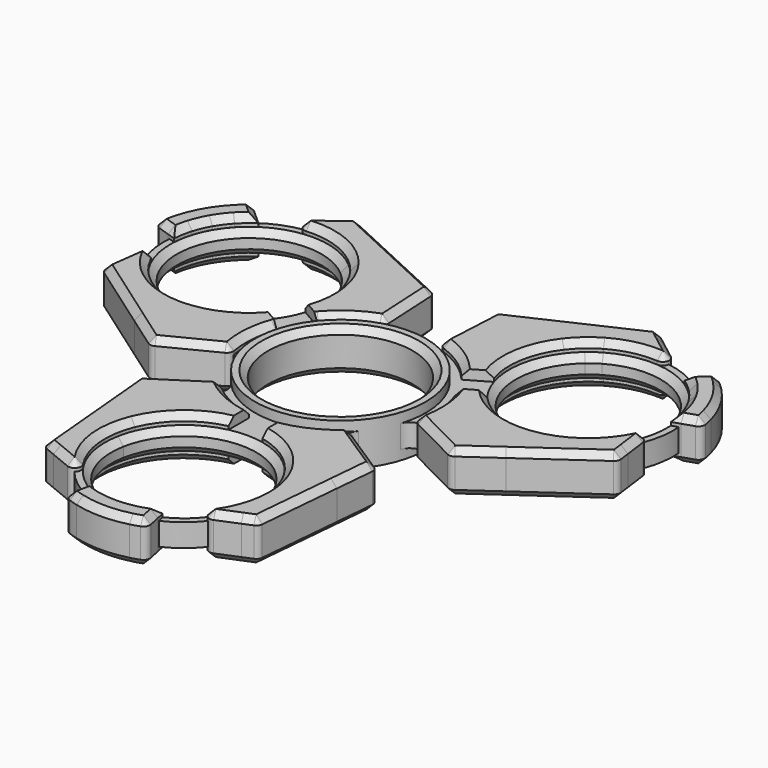
from build123d import *

# Parameters (mm, degrees)
F0_R         = 13.1
F0_R_2       = 11.1
F1_DEPTH     = 6.5
F3_DEPTH     = 6.5
F4_R         = 1
F4_2_R       = 1
F4_3_R       = 1
F6_SIZE      = 1
F6_2_SIZE    = 1
F6_3_SIZE    = 1
F6_4_SIZE    = 1
F7_COUNT     = 3
F10_DEPTH    = 3.5
F11_SIZE     = 1
F12_COUNT    = 3
F14_T1_DEPTH = 3.5


# Not quite as in the source:
# - a fillet or chamfer that OpenCascade refuses, or shapes differently, is made with other operations: its cross-section is extruded or revolved along the edge and cut away or added
# - two fillets or chamfers of one size are made in one step


with BuildPart() as f1:
    # F0 (on Top) → F1 (new body)
    with BuildSketch(Plane.XY):
        Circle(F0_R)
        Circle(F0_R_2, mode=Mode.SUBTRACT)
    extrude(amount=F1_DEPTH)

    # F6
    f6_edges = [f1.edges().sort_by_distance(p)[0] for p in [
        (-11.1, 0, 6.5),
        (-11.1, 0, 0),
    ]]
    chamfer(f6_edges, length=F6_SIZE)


with BuildPart() as f3:
    # F2 (on Top) → F3 (new body)
    with BuildSketch(Plane.XY):
        with BuildLine():
            Line((-14.7820725202, -23.8770650822), (-11.1789423434, -25.3695304684))
            ThreePointArc((-11.1789423434, -25.3695304684), (-7.7703064339, -20.7246381244), (-2.6, -18.1826398887))
            Line((-2.6, -18.1826398887), (-2.6, -14.2649921136))
            ThreePointArc((-2.6, -14.2649921136), (-2.6733155154, -14.2514344596), (-2.7465603489, -14.2375))
            ThreePointArc((-2.7465603489, -14.2375), (-10.0021770784, -17.5117473723), (-14.7820725202, -23.8770650822))
        make_face()
        with BuildLine():
            ThreePointArc((-6.2404261974, -40.3666330539), (-11.4929052715, -33.7845909184), (-11.1789423434, -25.3695304684))
            Line((-11.1789423434, -25.3695304684), (-14.7820725202, -23.8770650822))
            ThreePointArc((-14.7820725202, -23.8770650822), (-15.9929194856, -30.4759478198), (-14.3917986532, -36.9911466532))
            Line((-14.3917986532, -36.9911466532), (-6.2404261974, -40.3666330539))
        make_face()
        with BuildLine():
            Line((-17.6223396977, -22.7005878965), (-14.7820725202, -23.8770650822))
            ThreePointArc((-14.7820725202, -23.8770650822), (-10.0021770784, -17.5117473723), (-2.7465603489, -14.2375))
            ThreePointArc((-2.7465603489, -14.2375), (-6.5777497188, -12.9221982896), (-9.8956077284, -10.5984408139))
            Line((-9.8956077284, -10.5984408139), (-18.2283200336, -16.0097674569))
            Line((-18.2283200336, -16.0097674569), (-17.6223396977, -22.7005878965))
        make_face()
        with BuildLine():
            ThreePointArc((-14.3917986532, -36.9911466532), (-15.9929194856, -30.4759478198), (-14.7820725202, -23.8770650822))
            Line((-14.7820725202, -23.8770650822), (-17.6223396977, -22.7005878965))
            Line((-17.6223396977, -22.7005878965), (-16.4035077071, -36.1580971771))
            Line((-16.4035077071, -36.1580971771), (-14.3917986532, -36.9911466532))
        make_face()
    extrude(amount=F3_DEPTH)

    # F4#2
    f4_2_edges = [f3.edges().sort_by_distance(p)[0] for p in [
        (-6.240426, -40.366633, 3.25),
        (-9.895608, -10.598441, 3.25),
        (-18.22832, -16.009767, 3.25),
        (-16.403508, -36.158097, 3.25),
    ]]
    fillet(f4_2_edges, radius=F4_2_R)

    # F6#2
    f6_2_edges = [f3.edges().sort_by_distance(p)[0] for p in [
        (-11.248136, -25.540243, 6.5),
        (-11.248136, -25.540243, 0),
    ]]
    chamfer(f6_2_edges, length=F6_2_SIZE)


with BuildPart() as f3b:
    # F2 (on Top) → F3, piece 2 (new body)
    with BuildSketch(Plane.XY):
        with BuildLine():
            Line((14.7820725202, -23.8770650822), (11.1789423434, -25.3695304684))
            ThreePointArc((11.1789423434, -25.3695304684), (11.8675018929, -27.6394071036), (12.1, -30))
            ThreePointArc((12.1, -30), (10.5337352584, -35.9540256554), (6.2404261974, -40.3666330539))
            Line((6.2404261974, -40.3666330539), (14.3917986532, -36.9911466532))
            ThreePointArc((14.3917986532, -36.9911466532), (15.5927672087, -33.5868664283), (16, -30))
            ThreePointArc((16, -30), (15.6925644865, -26.8785548477), (14.7820725202, -23.8770650822))
        make_face()
        with BuildLine():
            Line((17.6223396977, -22.7005878965), (14.7820725202, -23.8770650822))
            ThreePointArc((14.7820725202, -23.8770650822), (15.6925644865, -26.8785548477), (16, -30))
            ThreePointArc((16, -30), (15.5927672087, -33.5868664283), (14.3917986532, -36.9911466532))
            Line((14.3917986532, -36.9911466532), (16.4035077071, -36.1580971771))
            Line((16.4035077071, -36.1580971771), (17.6223396977, -22.7005878965))
        make_face()
        with BuildLine():
            ThreePointArc((2.7465603489, -14.2375), (10.0021770784, -17.5117473723), (14.7820725202, -23.8770650822))
            Line((14.7820725202, -23.8770650822), (17.6223396977, -22.7005878965))
            Line((17.6223396977, -22.7005878965), (18.2283200336, -16.0097674569))
            Line((18.2283200336, -16.0097674569), (9.8956077284, -10.5984408139))
            ThreePointArc((9.8956077284, -10.5984408139), (6.5777497188, -12.9221982896), (2.7465603489, -14.2375))
        make_face()
        with BuildLine():
            ThreePointArc((2.6, -18.1826398887), (7.7703064339, -20.7246381244), (11.1789423434, -25.3695304684))
            Line((11.1789423434, -25.3695304684), (14.7820725202, -23.8770650822))
            ThreePointArc((14.7820725202, -23.8770650822), (10.0021770784, -17.5117473723), (2.7465603489, -14.2375))
            ThreePointArc((2.7465603489, -14.2375), (2.6733155154, -14.2514344596), (2.6, -14.2649921136))
            Line((2.6, -14.2649921136), (2.6, -18.1826398887))
        make_face()
    extrude(amount=F3_DEPTH)

    # F4#3
    f4_3_edges = [f3b.edges().sort_by_distance(p)[0] for p in [
        (6.240426, -40.366633, 3.25),
        (16.403508, -36.158097, 3.25),
        (18.22832, -16.009767, 3.25),
        (9.895608, -10.598441, 3.25),
    ]]
    fillet(f4_3_edges, radius=F4_3_R)

    # F6#3
    f6_3_edges = [f3b.edges().sort_by_distance(p)[0] for p in [
        (11.248136, -25.540243, 6.5),
        (11.248136, -25.540243, 0),
    ]]
    chamfer(f6_3_edges, length=F6_3_SIZE)


with BuildPart() as f3c:
    # F2 (on Top) → F3, piece 3 (new body)
    with BuildSketch(Plane.XY):
        with BuildLine():
            Line((2.8440204456, -42.1), (0, -42.1))
            Line((0, -42.1), (-2.8440204456, -42.1))
            Line((-2.8440204456, -42.1), (-4.0641319608, -45.4752328385))
            ThreePointArc((-4.0641319608, -45.4752328385), (0, -46), (4.0641319608, -45.4752328385))
            Line((4.0641319608, -45.4752328385), (2.8440204456, -42.1))
        make_face()
        with BuildLine():
            Line((-2.8440204456, -42.1), (0, -42.1))
            ThreePointArc((0, -42.1), (-1.3744675345, -42.0216820369), (-2.7311424248, -41.7877419829))
            Line((-2.7311424248, -41.7877419829), (-2.8440204456, -42.1))
        make_face()
        with BuildLine():
            ThreePointArc((2.7311424248, -41.7877419829), (1.3744675345, -42.0216820369), (0, -42.1))
            Line((0, -42.1), (2.8440204456, -42.1))
            Line((2.8440204456, -42.1), (2.7311424248, -41.7877419829))
        make_face()
        with BuildLine():
            Line((-4.0641319608, -45.4752328385), (-2.8440204456, -42.1))
            Line((-2.8440204456, -42.1), (-5.6838904288, -42.1))
            Line((-5.6838904288, -42.1), (-6.2404261974, -44.7328571864))
            ThreePointArc((-6.2404261974, -44.7328571864), (-5.1656325954, -45.1431912056), (-4.0641319608, -45.4752328385))
        make_face()
        with BuildLine():
            Line((5.6838904288, -42.1), (2.8440204456, -42.1))
            Line((2.8440204456, -42.1), (4.0641319608, -45.4752328385))
            ThreePointArc((4.0641319608, -45.4752328385), (5.1656325954, -45.1431912056), (6.2404261974, -44.7328571864))
            Line((6.2404261974, -44.7328571864), (5.6838904288, -42.1))
        make_face()
        with BuildLine():
            ThreePointArc((5.4136190846, -40.8214014068), (4.1009436156, -41.3838596909), (2.7311424248, -41.7877419829))
            Line((2.7311424248, -41.7877419829), (2.8440204456, -42.1))
            Line((2.8440204456, -42.1), (5.6838904288, -42.1))
            Line((5.6838904288, -42.1), (5.4136190846, -40.8214014068))
        make_face()
        with BuildLine():
            Line((-2.8440204456, -42.1), (-2.7311424248, -41.7877419829))
            ThreePointArc((-2.7311424248, -41.7877419829), (-4.1009436156, -41.3838596909), (-5.4136190846, -40.8214014068))
            Line((-5.4136190846, -40.8214014068), (-5.6838904288, -42.1))
            Line((-5.6838904288, -42.1), (-2.8440204456, -42.1))
        make_face()
    extrude(amount=F3_DEPTH)

    # F4
    f4_edges = [f3c.edges().sort_by_distance(p)[0] for p in [
        (-6.240426, -44.732857, 3.25),
        (6.240426, -44.732857, 3.25),
    ]]
    fillet(f4_edges, radius=F4_R)

    # F6#4
    f6_4_edges = [f3c.edges().sort_by_distance(p)[0] for p in [
        (0, -46, 0),
        (0, -46, 6.5),
        (0, -42.1, 6.5),
        (0, -42.1, 0),
    ]]
    chamfer(f6_4_edges, length=F6_4_SIZE)


with BuildPart() as f7_1:
    # F7: instance of F3c
    add(f3c.part.rotate(Axis((0, 0, 5.5), (0, 0, 1)), 1 * 360 / F7_COUNT))


with BuildPart() as f7_2:
    # F7: instance of F3c
    add(f3c.part.rotate(Axis((0, 0, 5.5), (0, 0, 1)), 2 * 360 / F7_COUNT))


with BuildPart() as f7_3:
    # F7: instance of F3
    add(f3.part.rotate(Axis((0, 0, 5.5), (0, 0, 1)), 1 * 360 / F7_COUNT))


with BuildPart() as f7_4:
    # F7: instance of F3
    add(f3.part.rotate(Axis((0, 0, 5.5), (0, 0, 1)), 2 * 360 / F7_COUNT))


with BuildPart() as f7_5:
    # F7: instance of F3b
    add(f3b.part.rotate(Axis((0, 0, 5.5), (0, 0, 1)), 1 * 360 / F7_COUNT))


with BuildPart() as f7_6:
    # F7: instance of F3b
    add(f3b.part.rotate(Axis((0, 0, 5.5), (0, 0, 1)), 2 * 360 / F7_COUNT))


with BuildPart() as f10:
    # F9 (on offset) → F10 (new body)
    with BuildSketch(Plane.XY.offset(1.5)):
        with BuildLine():
            ThreePointArc((-10.9083975794, -27.9465), (-11.8530394085, -27.5591265606), (-12.7839527001, -27.1398333333))
            ThreePointArc((-12.7839527001, -27.1398333333), (-1.4387876196, -43.0207484495), (13.1, -30))
            ThreePointArc((13.1, -30), (13.0207484495, -28.5612123804), (12.7839527001, -27.1398333333))
            ThreePointArc((12.7839527001, -27.1398333333), (11.8530394085, -27.5591265606), (10.9083975794, -27.9465))
            ThreePointArc((10.9083975794, -27.9465), (11.051995592, -28.9687903053), (11.1, -30))
            ThreePointArc((11.1, -30), (-1.0312096947, -41.051995592), (-10.9083975794, -27.9465))
        make_face()
        with BuildLine():
            ThreePointArc((-8.1424847512, -19.7379367534), (-11.0984667565, -23.0405434368), (-12.7839527001, -27.1398333333))
            ThreePointArc((-12.7839527001, -27.1398333333), (-11.8530394085, -27.5591265606), (-10.9083975794, -27.9465))
            ThreePointArc((-10.9083975794, -27.9465), (0, -18.9), (10.9083975794, -27.9465))
            ThreePointArc((10.9083975794, -27.9465), (11.8530394085, -27.5591265606), (12.7839527001, -27.1398333333))
            ThreePointArc((12.7839527001, -27.1398333333), (11.0984667565, -23.0405434368), (8.1424847512, -19.7379367534))
            ThreePointArc((8.1424847512, -19.7379367534), (0, -16.9), (-8.1424847512, -19.7379367534))
        make_face()
        with BuildLine():
            Line((-15.3728307724, -15.2988847025), (-8.1424847512, -19.7379367534))
            ThreePointArc((-8.1424847512, -19.7379367534), (0, -16.9), (8.1424847512, -19.7379367534))
            Line((8.1424847512, -19.7379367534), (15.3728307724, -15.2988847025))
            Line((15.3728307724, -15.2988847025), (7.8, -9.808))
            ThreePointArc((7.8, -9.808), (0, -12.5314350335), (-7.8, -9.808))
            Line((-7.8, -9.808), (-15.3728307724, -15.2988847025))
        make_face()
    extrude(amount=F10_DEPTH)

    # F11
    f11_edges = [f10.edges().sort_by_distance(p)[0] for p in [
        (-11.1, -30, 5),
        (-11.1, -30, 1.5),
    ]]
    chamfer(f11_edges, length=F11_SIZE)


with BuildPart() as f12_1:
    # F12: instance of F10
    add(f10.part.rotate(Axis((0, 0, 0), (0, 0, -1)), 1 * 360 / F12_COUNT))


with BuildPart() as f12_2:
    # F12: instance of F10
    add(f10.part.rotate(Axis((0, 0, 0), (0, 0, -1)), 2 * 360 / F12_COUNT))


with BuildPart() as f1_1:
    add(f1.part)

    # F13: union F3b, F3, F10, F12_1, F7_5, F7_3, F7_4, F12_2, F7_6
    add(f3b.part)
    add(f3.part)
    add(f10.part)
    add(f12_1.part)
    add(f7_5.part)
    add(f7_3.part)
    add(f7_4.part)
    add(f12_2.part)
    add(f7_6.part)

    # F14: fillet of radius 2 on 6 edges, made by hand

    # F14_s2 → F14_t1 (join)
    with BuildSketch(Plane.XY.offset(1.5)):
        with BuildLine():
            ThreePointArc((-9.7444700512, -8.7553014466), (-9.2486262566, -9.8359949684), (-9.4538478523, -11.007166883))
            Line((-9.4538478523, -11.007166883), (-9.4182813013, -11.0254704468))
            ThreePointArc((-9.4182813013, -11.0254704468), (-8.841949408, -10.6129017355), (-8.253531299, -10.1862533538))
            Line((-8.253531299, -10.1862533538), (-8.2517383163, -10.1228659361))
            ThreePointArc((-8.2517383163, -10.1228659361), (-9.010237875, -9.4540580406), (-9.7147159442, -8.7285677018))
            Line((-9.7147159442, -8.7285677018), (-9.7444700512, -8.7553014466))
        make_face()
        with BuildLine():
            ThreePointArc((9.7444700512, -8.7553014466), (9.2486262566, -9.8359949684), (9.4538478523, -11.007166883))
            Line((9.4538478523, -11.007166883), (9.4182813013, -11.0254704468))
            ThreePointArc((9.4182813013, -11.0254704468), (8.841949408, -10.6129017355), (8.253531299, -10.1862533538))
            Line((8.253531299, -10.1862533538), (8.2517383163, -10.1228659361))
            ThreePointArc((8.2517383163, -10.1228659361), (9.010237875, -9.4540580406), (9.7147159442, -8.7285677018))
            Line((9.7147159442, -8.7285677018), (9.7444700512, -8.7553014466))
        make_face()
        with BuildLine():
            ThreePointArc((2.710078445, 12.8166093341), (3.8939083859, 12.9275427725), (4.8055622182, 13.6908558451))
            Line((4.8055622182, 13.6908558451), (4.839196845, 13.6692060903))
            ThreePointArc((4.839196845, 13.6692060903), (4.7700678068, 12.9638036741), (4.6947885243, 12.2408944528))
            Line((4.6947885243, 12.2408944528), (4.6407899016, 12.2076479753))
            ThreePointArc((4.6407899016, 12.2076479753), (3.6823354945, 12.5301239142), (2.7018033963, 12.7774746491))
            Line((2.7018033963, 12.7774746491), (2.710078445, 12.8166093341))
        make_face()
        with BuildLine():
            ThreePointArc((-2.710078445, 12.8166093341), (-3.8939083859, 12.9275427725), (-4.8055622182, 13.6908558451))
            Line((-4.8055622182, 13.6908558451), (-4.839196845, 13.6692060903))
            ThreePointArc((-4.839196845, 13.6692060903), (-4.7700678068, 12.9638036741), (-4.6947885243, 12.2408944528))
            Line((-4.6947885243, 12.2408944528), (-4.6407899016, 12.2076479753))
            ThreePointArc((-4.6407899016, 12.2076479753), (-3.6823354945, 12.5301239142), (-2.7018033963, 12.7774746491))
            Line((-2.7018033963, 12.7774746491), (-2.710078445, 12.8166093341))
        make_face()
        with BuildLine():
            ThreePointArc((12.4545484962, -4.0613078874), (13.1425346425, -3.0915478041), (14.2594100705, -2.6836889621))
            Line((14.2594100705, -2.6836889621), (14.2574781463, -2.6437356435))
            ThreePointArc((14.2574781463, -2.6437356435), (13.6120172148, -2.3509019386), (12.9483198233, -2.0546410989))
            Line((12.9483198233, -2.0546410989), (12.8925282179, -2.0847820392))
            ThreePointArc((12.8925282179, -2.0847820392), (12.6925733695, -3.0760658736), (12.4165193405, -4.0489069473))
            Line((12.4165193405, -4.0489069473), (12.4545484962, -4.0613078874))
        make_face()
        with BuildLine():
            ThreePointArc((-12.4545484962, -4.0613078874), (-13.1425346425, -3.0915478041), (-14.2594100705, -2.6836889621))
            Line((-14.2594100705, -2.6836889621), (-14.2574781463, -2.6437356435))
            ThreePointArc((-14.2574781463, -2.6437356435), (-13.6120172148, -2.3509019386), (-12.9483198233, -2.0546410989))
            Line((-12.9483198233, -2.0546410989), (-12.8925282179, -2.0847820392))
            ThreePointArc((-12.8925282179, -2.0847820392), (-12.6925733695, -3.0760658736), (-12.4165193405, -4.0489069473))
            Line((-12.4165193405, -4.0489069473), (-12.4545484962, -4.0613078874))
        make_face()
    extrude(amount=F14_T1_DEPTH)


solid = Compound([f3c.part, f7_1.part, f7_2.part, f1_1.part])
